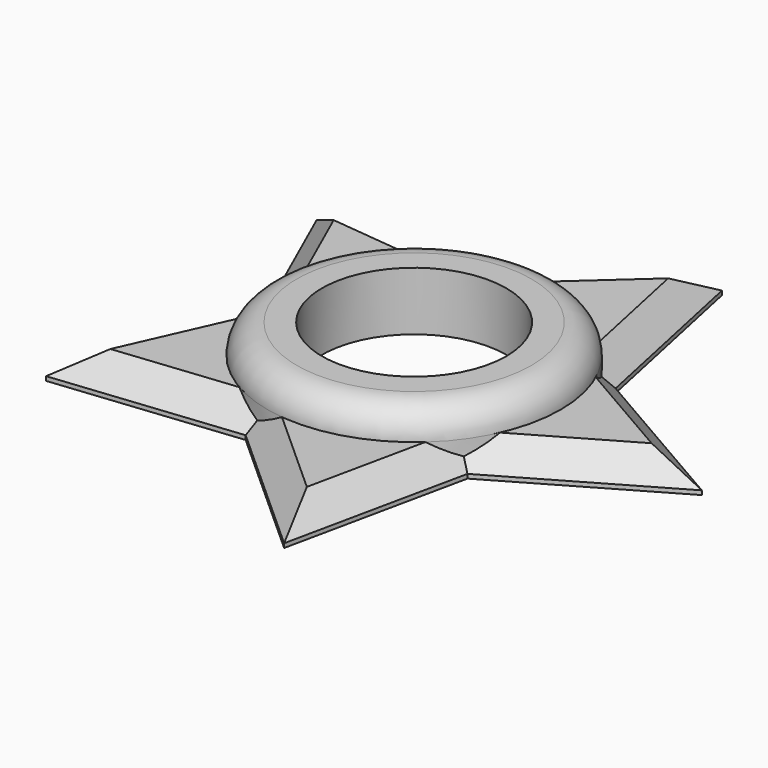
from build123d import *

# Parameters (mm, degrees)
F0_R          = 17.5
F0_R_2        = 11
F1_DEPTH      = 7
F3_DEPTH      = 3.5
F4_T4_DEPTH   = 37.5265318242
F4_T9_DEPTH   = 37.5265318242
F4_T14_DEPTH  = 37.5265318242
F4_T19_DEPTH  = 37.5265318242
F4_T24_DEPTH  = 37.5265318242
F4_T29_DEPTH  = 37.5265318242
F4_T34_DEPTH  = 37.5265318242
F4_T39_DEPTH  = 37.5265318242
F4_T44_DEPTH  = 37.5265318242
F4_T49_DEPTH  = 37.5265318242
F4_T55_DEPTH  = 37.5265318242
F4_S57_R      = 17.5
F4_T58_DEPTH  = 21
F4_T61_DEPTH  = 37.5265318242
F4_S63_R      = 17.5
F4_T64_DEPTH  = 22
F4_T70_DEPTH  = 37.5265318242
F4_S72_R      = 17.5
F4_T73_DEPTH  = 21
F4_T76_DEPTH  = 37.5265318242
F4_S78_R      = 17.5
F4_T79_DEPTH  = 22
F4_T85_DEPTH  = 37.5265318242
F4_S87_R      = 17.5
F4_T88_DEPTH  = 21
F4_T91_DEPTH  = 37.5265318242
F4_S93_R      = 17.5
F4_T94_DEPTH  = 22
F4_T100_DEPTH = 37.5265318242
F4_S102_R     = 17.5
F4_T103_DEPTH = 21
F4_T106_DEPTH = 37.5265318242
F4_S108_R     = 17.5
F4_T109_DEPTH = 21
F4_T115_DEPTH = 37.5265318242
F4_S117_R     = 17.5
F4_T118_DEPTH = 21
F4_T121_DEPTH = 37.5265318242
F4_S123_R     = 17.5
F4_T124_DEPTH = 22
F5_R          = 3.49999


# Not quite as in the source:
# - a fillet or chamfer that OpenCascade refuses, or shapes differently, is made with other operations: its cross-section is extruded or revolved along the edge and cut away or added
# - a fillet or chamfer is up to 0.001 mm smaller than in the source, because OpenCascade refuses the exact size


with BuildPart() as f1:
    # F0 (on Top) → F1 (new body)
    with BuildSketch(Plane.XY):
        Circle(F0_R)
        Circle(F0_R_2, mode=Mode.SUBTRACT)
    extrude(amount=F1_DEPTH)

    # F2 (on Top) → F3 (join)
    with BuildSketch(Plane.XY):
        Polygon((15.2065660609, 11.0482169482), (11.0207545101, 13.4648963738), (11.0207545101, 8.0070468423), (16.211477872, 6.3204785843), align=None)
        Polygon((11.0207545101, 8.0070468423), (11.0207545101, 13.4648963738), (15.2065660609, 11.0482169482), (10.6124591285, 32.6617907487), (-5.8083913831, 17.8763905373), (-1.0015101774, 17.3711669641), (-4.2095536412, 12.9556739404), align=None)
        Polygon((16.211477872, 6.3204785843), (11.0207545101, 8.0070468423), (11.0207545101, -8.0070468423), (16.211477872, -6.3204785843), (15.2065660609, -11.0482169482), (34.3426391482, 0), (15.2065660609, 11.0482169482), align=None)
        Polygon((16.211477872, -6.3204785843), (11.0207545101, -8.0070468423), (11.0207545101, -13.4648963738), (15.2065660609, -11.0482169482), align=None)
        Polygon((11.0207545101, -13.4648963738), (11.0207545101, -8.0070468423), (-4.2095536412, -12.9556739404), (-1.0015101774, -17.3711669641), (-5.8083913831, -17.8763905373), (10.6124591285, -32.6617907487), (15.2065660609, -11.0482169482), align=None)
        Polygon((-13.6224017379, 0), (-4.2095536412, 12.9556739404), (-9.4002770031, 14.6422421984), (-5.8083913831, 17.8763905373), (-27.7837787026, 20.1860968161), (-18.7963493557, 0), (-16.8304452017, 4.4154930237), align=None)
        Polygon((-9.4002770031, 14.6422421984), (-4.2095536412, 12.9556739404), (-1.0015101774, 17.3711669641), (-5.8083913831, 17.8763905373), align=None)
        Polygon((-9.4002770031, -14.6422421984), (-4.2095536412, -12.9556739404), (-13.6224017379, 0), (-16.8304452017, -4.4154930237), (-18.7963493557, 0), (-27.7837787026, -20.1860968161), (-5.8083913831, -17.8763905373), align=None)
        Polygon((-1.0015101774, -17.3711669641), (-4.2095536412, -12.9556739404), (-9.4002770031, -14.6422421984), (-5.8083913831, -17.8763905373), align=None)
        Polygon((-16.8304452017, -4.4154930237), (-13.6224017379, 0), (-16.8304452017, 4.4154930237), (-18.7963493557, 0), align=None)
    extrude(amount=F3_DEPTH)

    # F4: chamfer of 3 on 10 edges, made by hand


with BuildPart() as f4_tool2:
    # F4_s3 → F4_t4 (new body)
    with BuildSketch(Plane(origin=(0.0145298929, -0.0683577716, 0), x_dir=(0, 0, 1), z_dir=(-0.2079116908, 0.9781476007, 0))):
        Polygon((0.5, 17.1713195741), (3.5, 14.1713195741), (3.5, 17.1713195741), align=None)
    extrude(amount=F4_T4_DEPTH)

    split(bisect_by=Plane(origin=(8.5856597871, 14.8707989677, 0), x_dir=(0, 0, 1), z_dir=(0.5, 0.8660254038, 0)), keep=Keep.TOP)


with BuildPart() as f1_1:
    add(f1.part)

    # F4_t1: cut F4_tool2
    add(f4_tool2.part, mode=Mode.SUBTRACT)


with BuildPart() as f4_tool7:
    # F4_s8 → F4_t9 (new body)
    with BuildSketch(Plane(origin=(32.4384077554, -18.7283234496, 0), x_dir=(0, 0, 1), z_dir=(-0.8660254038, 0.5, 0))):
        Polygon((0.5, 17.1713195741), (3.5, 14.1713195741), (3.5, 17.1713195741), align=None)
    extrude(amount=F4_T9_DEPTH)

    split(bisect_by=Plane(origin=(16.7960850429, 3.5701180862, 0), x_dir=(0, 0, 1), z_dir=(0.9781476007, 0.2079116908, 0)), keep=Keep.TOP)


with BuildPart() as f1_2:
    add(f1_1.part)

    # F4_t6: cut F4_tool7
    add(f4_tool7.part, mode=Mode.SUBTRACT)


with BuildPart() as f4_tool12:
    # F4_s13 → F4_t14 (new body)
    with BuildSketch(Plane(origin=(-0.0605221203, -0.0349424625, 0), x_dir=(0, 0, 1), z_dir=(0.8660254038, 0.5, 0))):
        Polygon((0.5, 17.1713195741), (3.5, 14.1713195741), (3.5, 17.1713195741), align=None)
    extrude(amount=F4_T14_DEPTH)

    split(bisect_by=Plane(origin=(16.7960850429, -3.5701180862, 0), x_dir=(0, 0, 1), z_dir=(0.9781476007, -0.2079116908, 0)), keep=Keep.TOP)


with BuildPart() as f1_3:
    add(f1_2.part)

    # F4_t11: cut F4_tool12
    add(f4_tool12.part, mode=Mode.SUBTRACT)


with BuildPart() as f4_tool17:
    # F4_s18 → F4_t19 (new body)
    with BuildSketch(Plane(origin=(-7.7876747892, -36.6381292961, 0), x_dir=(0, 0, 1), z_dir=(0.2079116908, 0.9781476007, 0))):
        Polygon((0.5, 17.1713195741), (3.5, 14.1713195741), (3.5, 17.1713195741), align=None)
    extrude(amount=F4_T19_DEPTH)

    split(bisect_by=Plane(origin=(8.5856597871, -14.8707989677, 0), x_dir=(0, 0, 1), z_dir=(0.5, -0.8660254038, 0)), keep=Keep.TOP)


with BuildPart() as f1_4:
    add(f1_3.part)

    # F4_t16: cut F4_tool17
    add(f4_tool17.part, mode=Mode.SUBTRACT)


with BuildPart() as f4_tool22:
    # F4_s23 → F4_t24 (new body)
    with BuildSketch(Plane(origin=(-0.0519346203, 0.0467621422, 0), x_dir=(0, 0, 1), z_dir=(0.7431448255, -0.6691306064, 0))):
        Polygon((0.5, 17.1713195741), (3.5, 14.1713195741), (3.5, 17.1713195741), align=None)
    extrude(amount=F4_T24_DEPTH)

    split(bisect_by=Plane(origin=(1.7948916474, -17.0772532888, 0), x_dir=(0, 0, 1), z_dir=(0.1045284633, -0.9945218954, 0)), keep=Keep.TOP)


with BuildPart() as f1_5:
    add(f1_4.part)

    # F4_t21: cut F4_tool22
    add(f4_tool22.part, mode=Mode.SUBTRACT)


with BuildPart() as f4_tool27:
    # F4_s28 → F4_t29 (new body)
    with BuildSketch(Plane(origin=(-37.2514554684, -3.9152857395, 0), x_dir=(0, 0, 1), z_dir=(0.9945218954, 0.1045284633, 0))):
        Polygon((0.5, 17.1713195741), (3.5, 14.1713195741), (3.5, 17.1713195741), align=None)
    extrude(amount=F4_T29_DEPTH)

    split(bisect_by=Plane(origin=(-11.4898554786, -12.7607772881, 0), x_dir=(0, 0, 1), z_dir=(-0.6691306064, -0.7431448255, 0)), keep=Keep.TOP)


with BuildPart() as f1_6:
    add(f1_5.part)

    # F4_t26: cut F4_tool27
    add(f4_tool27.part, mode=Mode.SUBTRACT)


with BuildPart() as f4_tool32:
    # F4_s33 → F4_t34 (new body)
    with BuildSketch(Plane(origin=(0.0284247598, 0.0638430557, 0), x_dir=(0, 0, 1), z_dir=(-0.4067366431, -0.9135454576, 0))):
        Polygon((0.5, 17.1713195741), (3.5, 14.1713195741), (3.5, 17.1713195741), align=None)
    extrude(amount=F4_T34_DEPTH)

    split(bisect_by=Plane(origin=(-15.6867809987, -6.9842048808, 0), x_dir=(0, 0, 1), z_dir=(-0.9135454576, -0.4067366431, 0)), keep=Keep.TOP)


with BuildPart() as f1_7:
    add(f1_6.part)

    # F4_t31: cut F4_tool32
    add(f4_tool32.part, mode=Mode.SUBTRACT)


with BuildPart() as f4_tool37:
    # F4_s38 → F4_t39 (new body)
    with BuildSketch(Plane(origin=(-15.2349908207, 34.2183496334, 0), x_dir=(0, 0, 1), z_dir=(0.4067366431, -0.9135454576, 0))):
        Polygon((0.5, 17.1713195741), (3.5, 14.1713195741), (3.5, 17.1713195741), align=None)
    extrude(amount=F4_T39_DEPTH)

    split(bisect_by=Plane(origin=(-15.6867809987, 6.9842048808, 0), x_dir=(0, 0, 1), z_dir=(-0.9135454576, 0.4067366431, 0)), keep=Keep.TOP)


with BuildPart() as f1_8:
    add(f1_7.part)

    # F4_t36: cut F4_tool37
    add(f4_tool37.part, mode=Mode.SUBTRACT)


with BuildPart() as f4_tool42:
    # F4_s43 → F4_t44 (new body)
    with BuildSketch(Plane(origin=(0.069502088, -0.0073049638, 0), x_dir=(0, 0, 1), z_dir=(-0.9945218954, 0.1045284633, 0))):
        Polygon((0.5, 17.1713195741), (3.5, 14.1713195741), (3.5, 17.1713195741), align=None)
    extrude(amount=F4_T44_DEPTH)

    split(bisect_by=Plane(origin=(-11.4898554786, 12.7607772881, 0), x_dir=(0, 0, 1), z_dir=(-0.6691306064, 0.7431448255, 0)), keep=Keep.TOP)


with BuildPart() as f1_9:
    add(f1_8.part)

    # F4_t41: cut F4_tool42
    add(f4_tool42.part, mode=Mode.SUBTRACT)


with BuildPart() as f4_tool47:
    # F4_s48 → F4_t49 (new body)
    with BuildSketch(Plane(origin=(27.8357133229, 25.0633888519, 0), x_dir=(0, 0, 1), z_dir=(-0.7431448255, -0.6691306064, 0))):
        Polygon((0.5, 17.1713195741), (3.5, 14.1713195741), (3.5, 17.1713195741), align=None)
    extrude(amount=F4_T49_DEPTH)

    split(bisect_by=Plane(origin=(1.7948916474, 17.0772532888, 0), x_dir=(0, 0, 1), z_dir=(0.1045284633, 0.9945218954, 0)), keep=Keep.TOP)


with BuildPart() as f1_10:
    add(f1_9.part)

    # F4_t46: cut F4_tool47
    add(f4_tool47.part, mode=Mode.SUBTRACT)


with BuildPart() as f4_tool53:
    # F4_s54 → F4_t55 (new body)
    with BuildSketch(Plane(origin=(0.0145298929, -0.0683577716, 0), x_dir=(0, 0, 1), z_dir=(-0.2079116908, 0.9781476007, 0))):
        Polygon((0.5, 17.1713195741), (3.5, 14.1713195741), (3.5, 17.1713195741), align=None)
    extrude(amount=F4_T55_DEPTH)

    split(bisect_by=Plane(origin=(8.5856597871, 14.8707989677, 0), x_dir=(0, 0, 1), z_dir=(-0.5, -0.8660254038, 0)), keep=Keep.TOP)

    # F4_s57 → F4_t58 (cut, symmetric)
    with BuildSketch(Plane.XY.offset(2)):
        Circle(F4_S57_R)
    extrude(amount=F4_T58_DEPTH, both=True, mode=Mode.SUBTRACT)


with BuildPart() as f4_tool59:
    # F4_s60 → F4_t61 (new body)
    with BuildSketch(Plane(origin=(32.4384077554, -18.7283234496, 0), x_dir=(0, 0, 1), z_dir=(-0.8660254038, 0.5, 0))):
        Polygon((0.5, 17.1713195741), (3.5, 14.1713195741), (3.5, 17.1713195741), align=None)
    extrude(amount=F4_T61_DEPTH)

    split(bisect_by=Plane(origin=(16.7960850429, 3.5701180862, 0), x_dir=(0, 0, 1), z_dir=(-0.9781476007, -0.2079116908, 0)), keep=Keep.TOP)

    # F4_s63 → F4_t64 (cut, symmetric)
    with BuildSketch(Plane.XY.offset(2)):
        Circle(F4_S63_R)
    extrude(amount=F4_T64_DEPTH, both=True, mode=Mode.SUBTRACT)


with BuildPart() as f4_tool53_1:
    add(f4_tool53.part)

    # F4_t65: intersect F4_tool59
    add(f4_tool59.part, mode=Mode.INTERSECT)


with BuildPart() as f1_11:
    add(f1_10.part)

    # F4_t51: cut F4_tool53
    add(f4_tool53_1.part, mode=Mode.SUBTRACT)


with BuildPart() as f4_tool68:
    # F4_s69 → F4_t70 (new body)
    with BuildSketch(Plane(origin=(-7.7876747892, -36.6381292961, 0), x_dir=(0, 0, 1), z_dir=(0.2079116908, 0.9781476007, 0))):
        Polygon((0.5, 17.1713195741), (3.5, 14.1713195741), (3.5, 17.1713195741), align=None)
    extrude(amount=F4_T70_DEPTH)

    split(bisect_by=Plane(origin=(8.5856597871, -14.8707989677, 0), x_dir=(0, 0, 1), z_dir=(-0.5, 0.8660254038, 0)), keep=Keep.TOP)

    # F4_s72 → F4_t73 (cut, symmetric)
    with BuildSketch(Plane.XY.offset(2)):
        Circle(F4_S72_R)
    extrude(amount=F4_T73_DEPTH, both=True, mode=Mode.SUBTRACT)


with BuildPart() as f4_tool74:
    # F4_s75 → F4_t76 (new body)
    with BuildSketch(Plane(origin=(-0.0605221203, -0.0349424625, 0), x_dir=(0, 0, 1), z_dir=(0.8660254038, 0.5, 0))):
        Polygon((0.5, 17.1713195741), (3.5, 14.1713195741), (3.5, 17.1713195741), align=None)
    extrude(amount=F4_T76_DEPTH)

    split(bisect_by=Plane(origin=(16.7960850429, -3.5701180862, 0), x_dir=(0, 0, 1), z_dir=(-0.9781476007, 0.2079116908, 0)), keep=Keep.TOP)

    # F4_s78 → F4_t79 (cut, symmetric)
    with BuildSketch(Plane.XY.offset(2)):
        Circle(F4_S78_R)
    extrude(amount=F4_T79_DEPTH, both=True, mode=Mode.SUBTRACT)


with BuildPart() as f4_tool68_1:
    add(f4_tool68.part)

    # F4_t80: intersect F4_tool74
    add(f4_tool74.part, mode=Mode.INTERSECT)


with BuildPart() as f1_12:
    add(f1_11.part)

    # F4_t66: cut F4_tool68
    add(f4_tool68_1.part, mode=Mode.SUBTRACT)


with BuildPart() as f4_tool83:
    # F4_s84 → F4_t85 (new body)
    with BuildSketch(Plane(origin=(-37.2514554684, -3.9152857395, 0), x_dir=(0, 0, 1), z_dir=(0.9945218954, 0.1045284633, 0))):
        Polygon((0.5, 17.1713195741), (3.5, 14.1713195741), (3.5, 17.1713195741), align=None)
    extrude(amount=F4_T85_DEPTH)

    split(bisect_by=Plane(origin=(-11.4898554786, -12.7607772881, 0), x_dir=(0, 0, 1), z_dir=(0.6691306064, 0.7431448255, 0)), keep=Keep.TOP)

    # F4_s87 → F4_t88 (cut, symmetric)
    with BuildSketch(Plane.XY.offset(2)):
        Circle(F4_S87_R)
    extrude(amount=F4_T88_DEPTH, both=True, mode=Mode.SUBTRACT)


with BuildPart() as f4_tool89:
    # F4_s90 → F4_t91 (new body)
    with BuildSketch(Plane(origin=(-0.0519346203, 0.0467621422, 0), x_dir=(0, 0, 1), z_dir=(0.7431448255, -0.6691306064, 0))):
        Polygon((0.5, 17.1713195741), (3.5, 14.1713195741), (3.5, 17.1713195741), align=None)
    extrude(amount=F4_T91_DEPTH)

    split(bisect_by=Plane(origin=(1.7948916474, -17.0772532888, 0), x_dir=(0, 0, 1), z_dir=(-0.1045284633, 0.9945218954, 0)), keep=Keep.TOP)

    # F4_s93 → F4_t94 (cut, symmetric)
    with BuildSketch(Plane.XY.offset(2)):
        Circle(F4_S93_R)
    extrude(amount=F4_T94_DEPTH, both=True, mode=Mode.SUBTRACT)


with BuildPart() as f4_tool83_1:
    add(f4_tool83.part)

    # F4_t95: intersect F4_tool89
    add(f4_tool89.part, mode=Mode.INTERSECT)


with BuildPart() as f1_13:
    add(f1_12.part)

    # F4_t81: cut F4_tool83
    add(f4_tool83_1.part, mode=Mode.SUBTRACT)


with BuildPart() as f4_tool98:
    # F4_s99 → F4_t100 (new body)
    with BuildSketch(Plane(origin=(-15.2349908207, 34.2183496334, 0), x_dir=(0, 0, 1), z_dir=(0.4067366431, -0.9135454576, 0))):
        Polygon((0.5, 17.1713195741), (3.5, 14.1713195741), (3.5, 17.1713195741), align=None)
    extrude(amount=F4_T100_DEPTH)

    split(bisect_by=Plane(origin=(-15.6867809987, 6.9842048808, 0), x_dir=(0, 0, 1), z_dir=(0.9135454576, -0.4067366431, 0)), keep=Keep.TOP)

    # F4_s102 → F4_t103 (cut, symmetric)
    with BuildSketch(Plane.XY.offset(2)):
        Circle(F4_S102_R)
    extrude(amount=F4_T103_DEPTH, both=True, mode=Mode.SUBTRACT)


with BuildPart() as f4_tool104:
    # F4_s105 → F4_t106 (new body)
    with BuildSketch(Plane(origin=(0.0284247598, 0.0638430557, 0), x_dir=(0, 0, 1), z_dir=(-0.4067366431, -0.9135454576, 0))):
        Polygon((0.5, 17.1713195741), (3.5, 14.1713195741), (3.5, 17.1713195741), align=None)
    extrude(amount=F4_T106_DEPTH)

    split(bisect_by=Plane(origin=(-15.6867809987, -6.9842048808, 0), x_dir=(0, 0, 1), z_dir=(0.9135454576, 0.4067366431, 0)), keep=Keep.TOP)

    # F4_s108 → F4_t109 (cut, symmetric)
    with BuildSketch(Plane.XY.offset(2)):
        Circle(F4_S108_R)
    extrude(amount=F4_T109_DEPTH, both=True, mode=Mode.SUBTRACT)


with BuildPart() as f4_tool98_1:
    add(f4_tool98.part)

    # F4_t110: intersect F4_tool104
    add(f4_tool104.part, mode=Mode.INTERSECT)


with BuildPart() as f1_14:
    add(f1_13.part)

    # F4_t96: cut F4_tool98
    add(f4_tool98_1.part, mode=Mode.SUBTRACT)


with BuildPart() as f4_tool113:
    # F4_s114 → F4_t115 (new body)
    with BuildSketch(Plane(origin=(0.069502088, -0.0073049638, 0), x_dir=(0, 0, 1), z_dir=(-0.9945218954, 0.1045284633, 0))):
        Polygon((0.5, 17.1713195741), (3.5, 14.1713195741), (3.5, 17.1713195741), align=None)
    extrude(amount=F4_T115_DEPTH)

    split(bisect_by=Plane(origin=(-11.4898554786, 12.7607772881, 0), x_dir=(0, 0, 1), z_dir=(0.6691306064, -0.7431448255, 0)), keep=Keep.TOP)

    # F4_s117 → F4_t118 (cut, symmetric)
    with BuildSketch(Plane.XY.offset(2)):
        Circle(F4_S117_R)
    extrude(amount=F4_T118_DEPTH, both=True, mode=Mode.SUBTRACT)


with BuildPart() as f4_tool119:
    # F4_s120 → F4_t121 (new body)
    with BuildSketch(Plane(origin=(27.8357133229, 25.0633888519, 0), x_dir=(0, 0, 1), z_dir=(-0.7431448255, -0.6691306064, 0))):
        Polygon((0.5, 17.1713195741), (3.5, 14.1713195741), (3.5, 17.1713195741), align=None)
    extrude(amount=F4_T121_DEPTH)

    split(bisect_by=Plane(origin=(1.7948916474, 17.0772532888, 0), x_dir=(0, 0, 1), z_dir=(-0.1045284633, -0.9945218954, 0)), keep=Keep.TOP)

    # F4_s123 → F4_t124 (cut, symmetric)
    with BuildSketch(Plane.XY.offset(2)):
        Circle(F4_S123_R)
    extrude(amount=F4_T124_DEPTH, both=True, mode=Mode.SUBTRACT)


with BuildPart() as f4_tool113_1:
    add(f4_tool113.part)

    # F4_t125: intersect F4_tool119
    add(f4_tool119.part, mode=Mode.INTERSECT)


with BuildPart() as f1_15:
    add(f1_14.part)

    # F4_t111: cut F4_tool113
    add(f4_tool113_1.part, mode=Mode.SUBTRACT)

    # F5 (radius 3.5 in the source; OpenCascade refuses exactly that, so slightly less here)
    f5_edges = [f1_15.edges().sort_by_distance(p)[0] for p in [
        (-17.5, 0, 7),
    ]]
    fillet(f5_edges, radius=F5_R)


solid = f1_15.part
